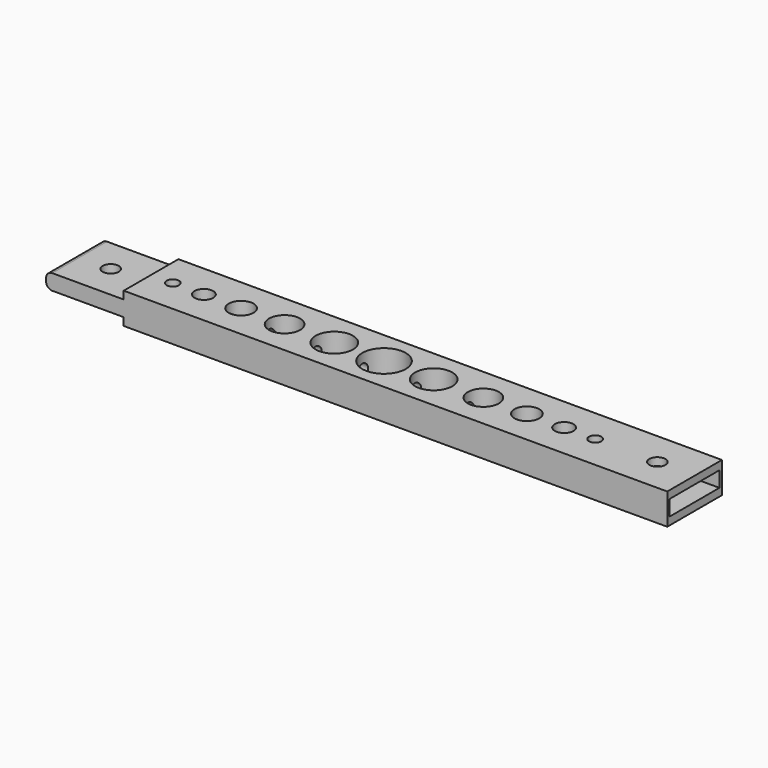
from build123d import *

# Parameters (mm, degrees)
F0_R      = 2
F0_R_2    = 3
F0_R_3    = 4
F0_R_4    = 5
F0_R_5    = 6
F0_R_6    = 7
F1_DEPTH  = 10
F2_START  = 2.5
F0_W      = 25
F0_H      = 22
F0_R_7    = 2.6
F2_DEPTH  = 5
F0_H_2    = 1
F0_H_3    = 20
F3_DEPTH  = 2.5
F4_DEPTH  = 10
F5_R      = 2
F6_R      = 2
F7_DEPTH  = 157.5
F8_R      = 2
F9_DEPTH  = 12
F10_DEPTH = 2.5
F11_START = 7.5
F11_DEPTH = 2.5


with BuildPart() as f1:
    # F0 (on Top) → F1 (new body)
    with BuildSketch(Plane.XY):
        Polygon((102.3076891899, 35.511040118), (-47.6923108101, 35.511040118), (-47.6923108101, 13.511040118), (102.3076891899, 13.511040118), (102.3076891899, 14.511040118), (102.3076891899, 34.511040118), align=None)
        with Locations((-40.6923108101, 24.511040118)):
            Circle(F0_R, mode=Mode.SUBTRACT)
        with Locations((-30.6923108101, 24.511040118)):
            Circle(F0_R_2, mode=Mode.SUBTRACT)
        with Locations((-18.6923108101, 24.511040118)):
            Circle(F0_R_3, mode=Mode.SUBTRACT)
        with Locations((-4.6923108101, 24.511040118)):
            Circle(F0_R_4, mode=Mode.SUBTRACT)
        with Locations((11.3076891899, 24.511040118)):
            Circle(F0_R_5, mode=Mode.SUBTRACT)
        with Locations((27.3076891899, 24.511040118)):
            Circle(F0_R_6, mode=Mode.SUBTRACT)
        with Locations((43.3076891899, 24.511040118)):
            Circle(F0_R_5, mode=Mode.SUBTRACT)
        with Locations((73.3076891899, 24.511040118)):
            Circle(F0_R_3, mode=Mode.SUBTRACT)
        with Locations((59.3076891899, 24.511040118)):
            Circle(F0_R_4, mode=Mode.SUBTRACT)
        with Locations((85.3076891899, 24.511040118)):
            Circle(F0_R_2, mode=Mode.SUBTRACT)
        with Locations((95.3076891899, 24.511040118)):
            Circle(F0_R, mode=Mode.SUBTRACT)
    extrude(amount=F1_DEPTH)

    # F0 (on Top) → F2 (join)
    with BuildSketch(Plane.XY.offset(F2_START)):
        with Locations((-60.1923108101, 24.511040118)):
            Rectangle(F0_W, F0_H)
        with Locations((-60.6923108101, 24.511040118)):
            Circle(F0_R_7, mode=Mode.SUBTRACT)
    extrude(amount=F2_DEPTH)

    # F0 (on Top) → F3 (join)
    with BuildSketch(Plane.XY):
        with Locations((114.8076891899, 35.011040118)):
            Rectangle(F0_W, F0_H_2)
        with Locations((114.8076891899, 24.511040118)):
            Rectangle(F0_W, F0_H_3)
        with Locations((115.3076891899, 24.511040118)):
            Circle(F0_R_7, mode=Mode.SUBTRACT)
        with Locations((114.8076891899, 14.011040118)):
            Rectangle(F0_W, F0_H_2)
    extrude(amount=F3_DEPTH)

    # F0 (on Top) → F4 (join)
    with BuildSketch(Plane.XY):
        with Locations((114.8076891899, 35.011040118)):
            Rectangle(F0_W, F0_H_2)
        with Locations((114.8076891899, 14.011040118)):
            Rectangle(F0_W, F0_H_2)
    extrude(amount=F4_DEPTH)

    # F5
    f5_edges = [f1.edges().sort_by_distance(p)[0] for p in [
        (-72.692311, 24.51104, 7.5),
        (-72.692311, 24.51104, 2.5),
    ]]
    fillet(f5_edges, radius=F5_R)

    # F6 (on face) → F7 (cut)
    with BuildSketch(Plane.YZ.offset(102.3076891899)):
        with Locations((24.511040118, 5)):
            Circle(F6_R)
    extrude(amount=-F7_DEPTH, mode=Mode.SUBTRACT)

    # F8 (on face) → F9 (cut)
    with BuildSketch(Plane(origin=(0, 35.511040118, 0), x_dir=(-1, 0, 0), z_dir=(0, 1, 0))):
        with Locations((52.6923108101, 5)):
            Circle(F8_R)
    extrude(amount=-F9_DEPTH, mode=Mode.SUBTRACT)

    # F0 (on Top) → F10 (join)
    with BuildSketch(Plane.XY):
        with Locations((114.8076891899, 24.511040118)):
            Rectangle(F0_W, F0_H_3)
        with Locations((115.3076891899, 24.511040118)):
            Circle(F0_R_7, mode=Mode.SUBTRACT)
    extrude(amount=F10_DEPTH)

    # F0 (on Top) → F11 (join)
    with BuildSketch(Plane.XY.offset(F11_START)):
        with Locations((114.8076891899, 24.511040118)):
            Rectangle(F0_W, F0_H_3)
        with Locations((115.3076891899, 24.511040118)):
            Circle(F0_R_7, mode=Mode.SUBTRACT)
    extrude(amount=F11_DEPTH)


solid = f1.part
